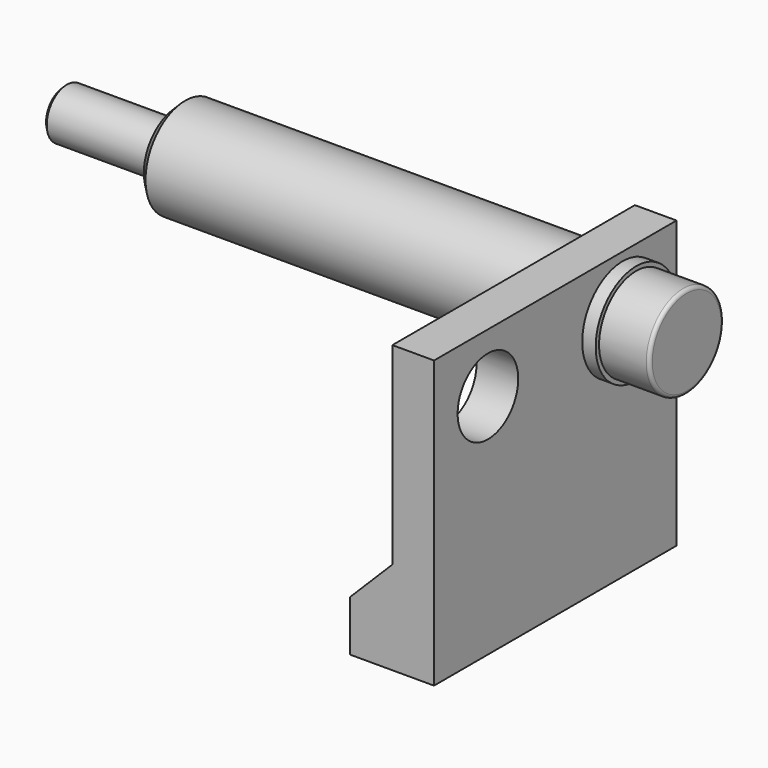
from build123d import *

# Parameters (mm, degrees)
F1_DEPTH  = 9
F3_D      = 4.5
F4_R      = 2.95
F5_DEPTH  = 24
F6_R      = 2.15
F7_DEPTH  = 2.3
F8_SIZE   = 0.5
F9_SIZE   = 0.5
F11_D     = 3.2
F12_R     = 3
F12_R_2   = 1.6
F13_DEPTH = 0.8
F14_R     = 1.5
F15_DEPTH = 34
F16_R     = 2.75
F17_DEPTH = 3
F18_R     = 0.2
F19_SIZE  = 0.2


with BuildPart() as f1:
    # F0 (on Front) → F1 (new body, symmetric)
    with BuildSketch(Plane.XZ):
        Polygon((10.6045, -3.0607), (8.7843067812, -4.8808932188), (8.7843067812, -7.8808932188), (13.7843067812, -7.8808932188), (13.7843067812, 9.1191067812), (11.3116067812, 9.1191067812), (11.3116067812, -2.3535932188), align=None)
    extrude(amount=F1_DEPTH, both=True)

    # F3 (through all)
    with Locations(Plane.YZ.offset(13.7843067812)):
        with Locations((-5, 5.6191067812), (5, 5.6191067812)):
            Hole(F3_D / 2)


with BuildPart() as f5:
    # F4 (on face) → F5 (new body)
    with BuildSketch(Plane(origin=(11.3116067812, 0, 0), x_dir=(0, -1, 0), z_dir=(-1, 0, 0))):
        with Locations((-5, 5.6191067812)):
            Circle(F4_R)
    extrude(amount=F5_DEPTH)

    # F6 (on face) → F7 (join)
    with BuildSketch(Plane.YZ.offset(11.3116067812)):
        with Locations((5, 5.6191067812)):
            Circle(F6_R)
    extrude(amount=F7_DEPTH)

    # F8
    f8_edges = [f5.edges().sort_by_distance(p)[0] for p in [
        (13.611607, 2.85, 5.619107),
    ]]
    chamfer(f8_edges, length=F8_SIZE)

    # F9
    f9_edges = [f5.edges().sort_by_distance(p)[0] for p in [
        (-12.688393, 7.95, 5.619107),
    ]]
    chamfer(f9_edges, length=F9_SIZE)

    # F11 (through all)
    with Locations(Plane.YZ.offset(13.6116067812)):
        with Locations((5, 5.6191067812)):
            Hole(F11_D / 2)


with BuildPart() as f13:
    # F12 (on face) → F13 (new body)
    with BuildSketch(Plane.YZ.offset(13.7843067812)):
        with Locations((5, 5.6191067812)):
            Circle(F12_R)
        with Locations((5, 5.6191067812)):
            Circle(F12_R_2, mode=Mode.SUBTRACT)
    extrude(amount=F13_DEPTH)


with BuildPart() as f15:
    # F14 (on face) → F15 (new body)
    with BuildSketch(Plane.YZ.offset(14.5843067812)):
        with Locations((5, 5.6191067812)):
            Circle(F14_R)
    extrude(amount=-F15_DEPTH)

    # F16 (on face) → F17 (join)
    with BuildSketch(Plane.YZ.offset(14.5843067812)):
        with Locations((5, 5.6191067812)):
            Circle(F16_R)
    extrude(amount=F17_DEPTH)

    # F18
    f18_edges = [f15.edges().sort_by_distance(p)[0] for p in [
        (17.584307, 2.25, 5.619107),
        (14.584307, 3.5, 5.619107),
    ]]
    fillet(f18_edges, radius=F18_R)

    # F19
    f19_edges = [f15.edges().sort_by_distance(p)[0] for p in [
        (-19.415693, 3.5, 5.619107),
    ]]
    chamfer(f19_edges, length=F19_SIZE)


solid = Compound([f1.part, f5.part, f13.part, f15.part])
